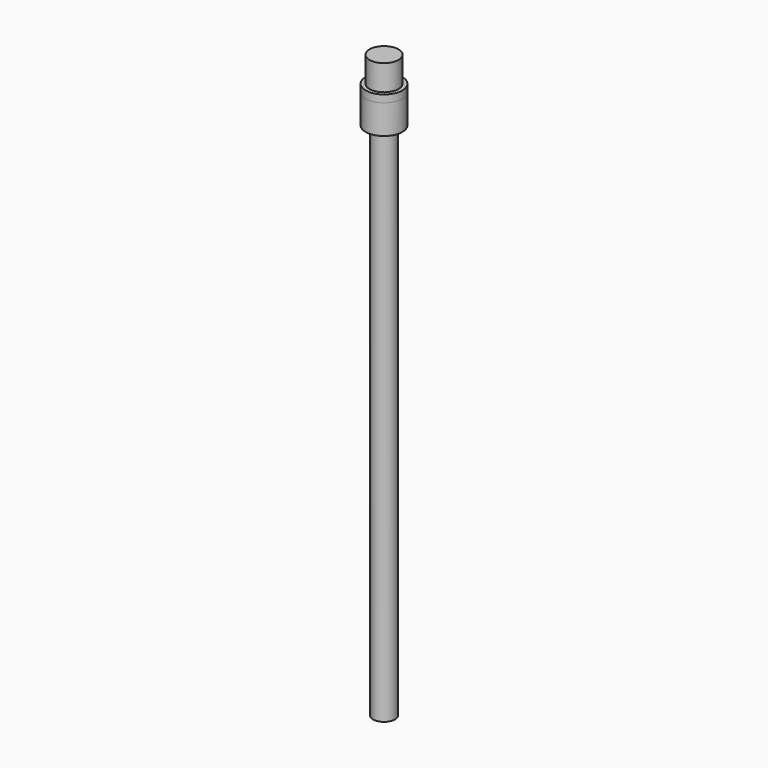
from build123d import *

# Parameters (mm, degrees)
F0_R     = 3
F1_DEPTH = 150
F2_R     = 5
F2_R_2   = 3
F3_DEPTH = 8
F4_DEPTH = 2
F5_R     = 3.95
F6_DEPTH = 7


with BuildPart() as f1:
    # F0 (on Top) → F1 (new body)
    with BuildSketch(Plane.XY):
        Circle(F0_R)
    extrude(amount=F1_DEPTH)


with BuildPart() as f3:
    # F2 (on face) → F3 (new body)
    with BuildSketch(Plane.XY.offset(150)):
        Circle(F2_R)
        Circle(F2_R_2, mode=Mode.SUBTRACT)
    extrude(amount=-F3_DEPTH)

    # F2 (on face) → F4 (join)
    with BuildSketch(Plane.XY.offset(150)):
        Circle(F2_R)
        Circle(F2_R_2, mode=Mode.SUBTRACT)
        Circle(F2_R_2)
    extrude(amount=F4_DEPTH)

    # F5 (on face) → F6 (join)
    with BuildSketch(Plane.XY.offset(152)):
        Circle(F5_R)
    extrude(amount=F6_DEPTH)


solid = Compound([f1.part, f3.part])
